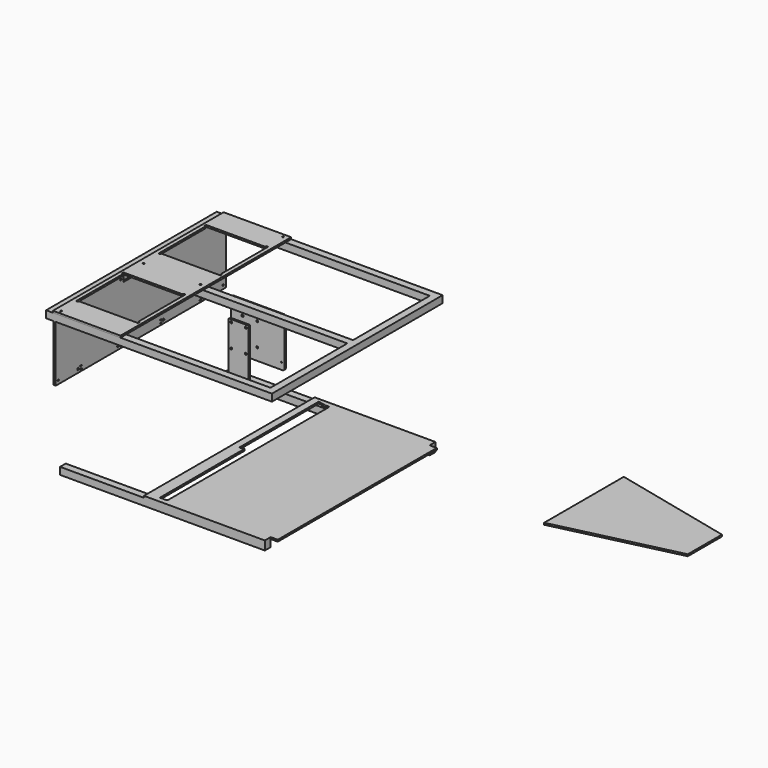
from build123d import *

# Parameters (mm, degrees)
F2_R      = 1.4
F2_W      = 5.1
F2_H      = 5.1
F3_DEPTH  = 5
F0_R      = 1.4
F0_W      = 5.1
F0_H      = 5.1
F0_R_2    = 2.25
F4_DEPTH  = 5
F9_W      = 595.277
F9_H      = 20
F9_W_2    = 20
F10_DEPTH = 20
F11_DEPTH = 5
F13_W     = 20
F13_H     = 20
F14_DEPTH = 576
F15_R     = 2.25
F15_W     = 6
F15_H     = 2
F15_R_2   = 3
F16_DEPTH = 5
F17_R     = 2.25
F18_DEPTH = 5


with BuildPart() as f3:
    # F2 (on offset) → F3 (new body)
    with BuildSketch(Plane.XZ.offset(35)):
        with BuildLine():
            ThreePointArc((-28, 2), (-27.4142135624, 0.5857864376), (-26, 0))
            Line((-26, 0), (-22, 0))
            ThreePointArc((-22, 0), (-20.5857864376, 0.5857864376), (-20, 2))
            Line((-20, 2), (-20, 11))
            Line((-20, 11), (20, 11))
            Line((20, 11), (20, 2))
            ThreePointArc((20, 2), (20.5857864376, 0.5857864376), (22, 0))
            Line((22, 0), (26, 0))
            ThreePointArc((26, 0), (27.4142135624, 0.5857864376), (28, 2))
            Line((28, 2), (28, 163))
            ThreePointArc((28, 163), (27.4142135624, 164.4142135624), (26, 165))
            Line((26, 165), (-26, 165))
            ThreePointArc((-26, 165), (-27.4142135624, 164.4142135624), (-28, 163))
            Line((-28, 163), (-28, 2))
        make_face()
        with Locations((-24, 5)):
            Circle(F2_R, mode=Mode.SUBTRACT)
        with Locations((24, 5)):
            Circle(F2_R, mode=Mode.SUBTRACT)
        with Locations((-20.5, 92.5)):
            Rectangle(F2_W, F2_H, mode=Mode.SUBTRACT)
        with Locations((-20.5, 157.5)):
            Rectangle(F2_W, F2_H, mode=Mode.SUBTRACT)
        with Locations((20.5, 92.5)):
            Rectangle(F2_W, F2_H, mode=Mode.SUBTRACT)
        with Locations((20.5, 157.5)):
            Rectangle(F2_W, F2_H, mode=Mode.SUBTRACT)
    extrude(amount=F3_DEPTH)


with BuildPart() as f4:
    # F0 (on Front) → F4 (new body)
    with BuildSketch(Plane.XZ):
        with BuildLine():
            Line((-53, 191), (-53, 64))
            ThreePointArc((-53, 64), (-51.5355339059, 60.4644660941), (-48, 59))
            Line((-48, 59), (92, 59))
            ThreePointArc((92, 59), (95.5355339059, 60.4644660941), (97, 64))
            Line((97, 64), (97, 191))
            ThreePointArc((97, 191), (95.5355339059, 194.5355339059), (92, 196))
            Line((92, 196), (-48, 196))
            ThreePointArc((-48, 196), (-51.5355339059, 194.5355339059), (-53, 191))
        make_face()
        with Locations((-45, 67)):
            Circle(F0_R, mode=Mode.SUBTRACT)
        with Locations((-20.5, 92.5)):
            Rectangle(F0_W, F0_H, mode=Mode.SUBTRACT)
        with Locations((20.5, 92.5)):
            Rectangle(F0_W, F0_H, mode=Mode.SUBTRACT)
        with Locations((89, 78)):
            Circle(F0_R, mode=Mode.SUBTRACT)
        with Locations((-20.5, 157.5)):
            Rectangle(F0_W, F0_H, mode=Mode.SUBTRACT)
        with Locations((20.5, 157.5)):
            Rectangle(F0_W, F0_H, mode=Mode.SUBTRACT)
        with Locations((-45, 188)):
            Circle(F0_R_2, mode=Mode.SUBTRACT)
        with Locations((89, 188)):
            Circle(F0_R_2, mode=Mode.SUBTRACT)
    extrude(amount=-F4_DEPTH)

    # F9 (on offset) → F10 (join)
    with BuildSketch(Plane.XY.offset(178)):
        with Locations((-7.6385, 280)):
            Rectangle(F9_W, F9_H)
        Polygon((-305.277, 0), (-305.277, 270), (-325.277, 270), (-325.277, -290), (-305.277, -290), (-305.277, -20), align=None)
        with Locations((-315.277, 280)):
            Rectangle(F9_W_2, F9_H)
        Polygon((310, 270), (290, 270), (290, 0), (290, -20), (290, -290), (310, -290), align=None)
        with Locations((300, 280)):
            Rectangle(F9_W_2, F9_H)
        with Locations((-315.277, -300)):
            Rectangle(F9_W_2, F9_H)
        with Locations((300, -300)):
            Rectangle(F9_W_2, F9_H)
        with Locations((-7.6385, -300)):
            Rectangle(F9_W, F9_H)
        with Locations((-7.6385, -10)):
            Rectangle(F9_W, F9_H)
    extrude(amount=F10_DEPTH)


with BuildPart() as f11:
    # F7 (on offset) → F11 (new body)
    with BuildSketch(Plane.XY.offset(-172)):
        with BuildLine():
            Line((290, 269.5), (290, 290))
            Line((290, 290), (-50, 290))
            Line((-50, 290), (-50, -310))
            Line((-50, -310), (290, -310))
            Line((290, -310), (290, -289.5))
            Line((290, -289.5), (310, -289.5))
            Line((310, -289.5), (310, 80))
            Line((310, 80), (3.839, 7.9621176471))
            Line((3.839, 7.9621176471), (3.839, -54.7018833458))
            Line((3.839, -54.7018833458), (3.839, -292))
            ThreePointArc((3.839, -292), (2.9603203436, -294.1213203436), (0.839, -295))
            Line((0.839, -295), (-12.161, -295))
            Line((-12.161, -295), (-17.161, -295))
            Line((-17.161, -295), (-17.161, -54.9885779619))
            Line((-17.161, -54.9885779619), (-17.161, 3.0209411765))
            Line((-17.161, 3.0209411765), (-30, 0))
            Line((-30, 0), (-30, 280))
            Line((-30, 280), (-8.75, 275))
            Line((-8.75, 275), (0.839, 275))
            ThreePointArc((0.839, 275), (2.9468642744, 274.1346915938), (3.8387600983, 272.0379388004))
            Line((3.8387600983, 272.0379388004), (310, 200))
            Line((310, 200), (310, 269.5))
            Line((310, 269.5), (290, 269.5))
        make_face()
        with BuildLine():
            Line((310, 80), (310, 200))
            Line((310, 200), (3.8387600983, 272.0379388004))
            ThreePointArc((3.8387600983, 272.0379388004), (3.838940024, 272.0189697794), (3.839, 272))
            Line((3.839, 272), (3.839, 16.7615581304))
            Line((3.839, 16.7615581304), (3.839, 7.9621176471))
            Line((3.839, 7.9621176471), (310, 80))
        make_face()
    extrude(amount=-F11_DEPTH)

    # F13 (on face) → F14 (join)
    with BuildSketch(Plane.YZ.offset(290)):
        with Locations((-300, -187)):
            Rectangle(F13_W, F13_H)
        with Locations((280, -187)):
            Rectangle(F13_W, F13_H)
    extrude(amount=-F14_DEPTH)


with BuildPart() as f11b:
    # F7 (on offset) → F11, piece 2 (new body)
    with BuildSketch(Plane.XY.offset(-172)):
        Polygon((1056.4796590805, 339.0180289745), (716.4796590805, 419.0180289745), (716.4796590805, 139.0180289745), (1056.4796590805, 219.0180289745), align=None)
    extrude(amount=-F11_DEPTH)


with BuildPart() as f16:
    # F15 (on face) → F16 (new body)
    with BuildSketch(Plane.YZ.offset(-305.277)):
        with BuildLine():
            ThreePointArc((-308.5, 20.0000003302), (-307.9142135624, 18.5857867678), (-306.5, 18.0000003302))
            Line((-306.5, 18.0000003302), (289.5, 18.0000003302))
            ThreePointArc((289.5, 18.0000003302), (290.9142135624, 18.5857867678), (291.5, 20.0000003302))
            Line((291.5, 20.0000003302), (291.5, 178.0000003302))
            Line((291.5, 178.0000003302), (271, 178.0000003302))
            Line((271, 178.0000003302), (271, 198.0000003302))
            Line((271, 198.0000003302), (51.5, 198.0000003302))
            Line((51.5, 198.0000003302), (51.5, 178.0000003302))
            Line((51.5, 178.0000003302), (-68.5, 178.0000003302))
            Line((-68.5, 178.0000003302), (-68.5, 198.0000003302))
            Line((-68.5, 198.0000003302), (-288, 198.0000003302))
            Line((-288, 198.0000003302), (-288, 178.0000003302))
            Line((-288, 178.0000003302), (-308.5, 178.0000003302))
            Line((-308.5, 178.0000003302), (-308.5, 20.0000003302))
        make_face()
        with Locations((-298.5, 28.0000003302)):
            Circle(F15_R, mode=Mode.SUBTRACT)
        with Locations((-218.5, 23.5000003302)):
            Rectangle(F15_W, F15_H, mode=Mode.SUBTRACT)
        with Locations((-228.5, 27.5000003302)):
            Circle(F15_R_2, mode=Mode.SUBTRACT)
        with Locations((-218.5, 31.5000003302)):
            Rectangle(F15_W, F15_H, mode=Mode.SUBTRACT)
        with Locations((-88.5, 27.5000003302)):
            Circle(F15_R_2, mode=Mode.SUBTRACT)
        with Locations((-78.5, 23.5000003302)):
            Rectangle(F15_W, F15_H, mode=Mode.SUBTRACT)
        with Locations((-78.5, 31.5000003302)):
            Rectangle(F15_W, F15_H, mode=Mode.SUBTRACT)
        with Locations((61.5, 23.5000003302)):
            Rectangle(F15_W, F15_H, mode=Mode.SUBTRACT)
        with Locations((61.5, 31.5000003302)):
            Rectangle(F15_W, F15_H, mode=Mode.SUBTRACT)
        with Locations((71.5, 27.5000003302)):
            Circle(F15_R_2, mode=Mode.SUBTRACT)
        with Locations((201.5, 23.5000003302)):
            Rectangle(F15_W, F15_H, mode=Mode.SUBTRACT)
        with Locations((211.5, 27.5000003302)):
            Circle(F15_R_2, mode=Mode.SUBTRACT)
        with Locations((201.5, 31.5000003302)):
            Rectangle(F15_W, F15_H, mode=Mode.SUBTRACT)
        with Locations((281.5, 28.0000003302)):
            Circle(F15_R, mode=Mode.SUBTRACT)
        with Locations((-78.5, 188.0000003302)):
            Circle(F15_R, mode=Mode.SUBTRACT)
    extrude(amount=F16_DEPTH)


with BuildPart() as f18:
    # F17 (on face) → F18 (new body)
    with BuildSketch(Plane.XY.offset(198)):
        Polygon((-306, 290), (-306, -20), (-211, -20), (-211, 0), (-116, 0), (-116, 290), align=None)
        with Locations((-291, -10)):
            Circle(F17_R, mode=Mode.SUBTRACT)
        Polygon((-295, 47.5), (-295, 51), (-295, 213.5), (-298.5, 213.5), (-298.5, 219), (-295, 219), (-132.5, 219), (-132.5, 222.5), (-127, 222.5), (-127, 219), (-127, 56.5), (-123.5, 56.5), (-123.5, 51), (-127, 51), (-289.5, 51), (-289.5, 47.5), align=None, mode=Mode.SUBTRACT)
        with Locations((-131, 280)):
            Circle(F17_R, mode=Mode.SUBTRACT)
        Polygon((-211, -20), (-306, -20), (-306, -310), (-116, -310), (-116, 0), (-211, 0), align=None)
        with Locations((-291, -300)):
            Circle(F17_R, mode=Mode.SUBTRACT)
        Polygon((-295, -71), (-132.5, -71), (-132.5, -67.5), (-127, -67.5), (-127, -71), (-127, -233.5), (-123.5, -233.5), (-123.5, -239), (-127, -239), (-289.5, -239), (-289.5, -242.5), (-295, -242.5), (-295, -239), (-295, -76.5), (-298.5, -76.5), (-298.5, -71), align=None, mode=Mode.SUBTRACT)
        with Locations((-131, -10)):
            Circle(F17_R, mode=Mode.SUBTRACT)
    extrude(amount=F18_DEPTH)


solid = Compound([f3.part, f4.part, f11.part, f11b.part, f16.part, f18.part])
